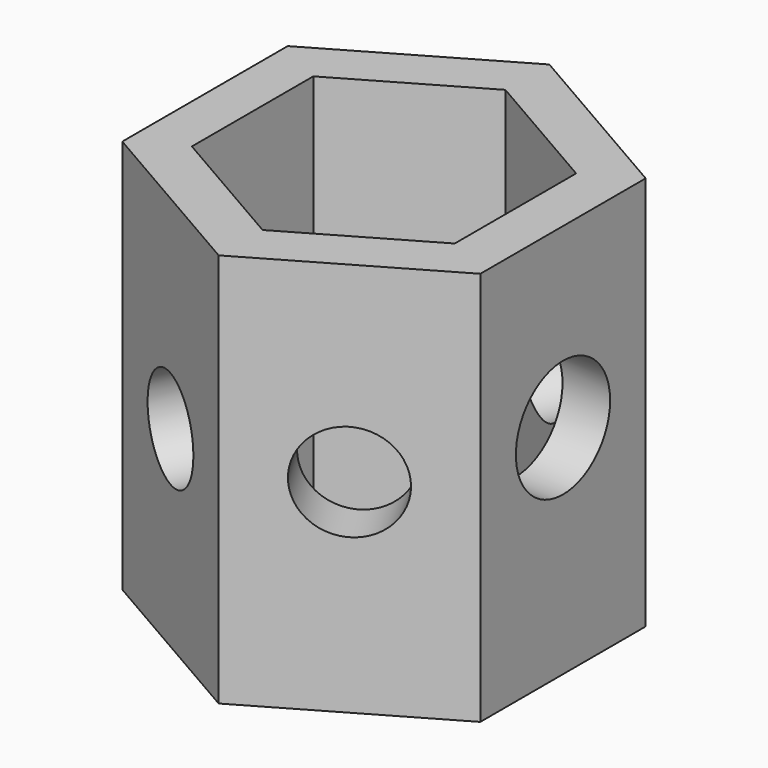
from build123d import *

# Parameters (mm, degrees)
F1_DEPTH = 50.8
F2_R     = 7.58365402
F3_DEPTH = 38.1
F4_DEPTH = 38.1
F5_R     = 6.3202279554
F6_DEPTH = 76.2
F7_R     = 6.2629522454
F8_DEPTH = 50.8


with BuildPart() as f1:
    # F0 (on Top) → F1 (new body)
    with BuildSketch(Plane.XY):
        Polygon((-23.0499133468, 13.3078736756), (-23.0499133468, -13.3078736756), (0, -26.6157473511), (23.0499133468, -13.3078736756), (23.0499133468, 13.3078736756), (0, 26.6157473511), align=None)
        Polygon((0, -19.5391465708), (-16.9213972986, -9.7695732854), (-16.9213972986, 9.7695732854), (0, 19.5391465708), (16.9213972986, 9.7695732854), (16.9213972986, -9.7695732854), align=None, mode=Mode.SUBTRACT)
    extrude(amount=F1_DEPTH)

    # F2 (on Right) → F3 (cut)
    with BuildSketch(Plane.YZ):
        with Locations((0, 27.9511734843)):
            Circle(F2_R)
    extrude(amount=F3_DEPTH, mode=Mode.SUBTRACT)

    # F2 (on Right) → F4 (cut)
    with BuildSketch(Plane.YZ):
        with Locations((0, 27.9511734843)):
            Circle(F2_R)
    extrude(amount=-F4_DEPTH, mode=Mode.SUBTRACT)

    # F5 (on face) → F6 (cut)
    with BuildSketch(Plane(origin=(-11.5249566734, -19.9618105133, 0), x_dir=(0.8660254038, -0.5, 0), z_dir=(-0.5, -0.8660254038, 0))):
        with Locations((0, 24.6956739575)):
            Circle(F5_R)
    extrude(amount=-F6_DEPTH, mode=Mode.SUBTRACT)

    # F7 (on face) → F8 (cut)
    with BuildSketch(Plane(origin=(11.5249566734, -19.9618105133, 0), x_dir=(0.8660254038, 0.5, 0), z_dir=(0.5, -0.8660254038, 0))):
        with Locations((0, 26.1488687247)):
            Circle(F7_R)
    extrude(amount=-F8_DEPTH, mode=Mode.SUBTRACT)


solid = f1.part
